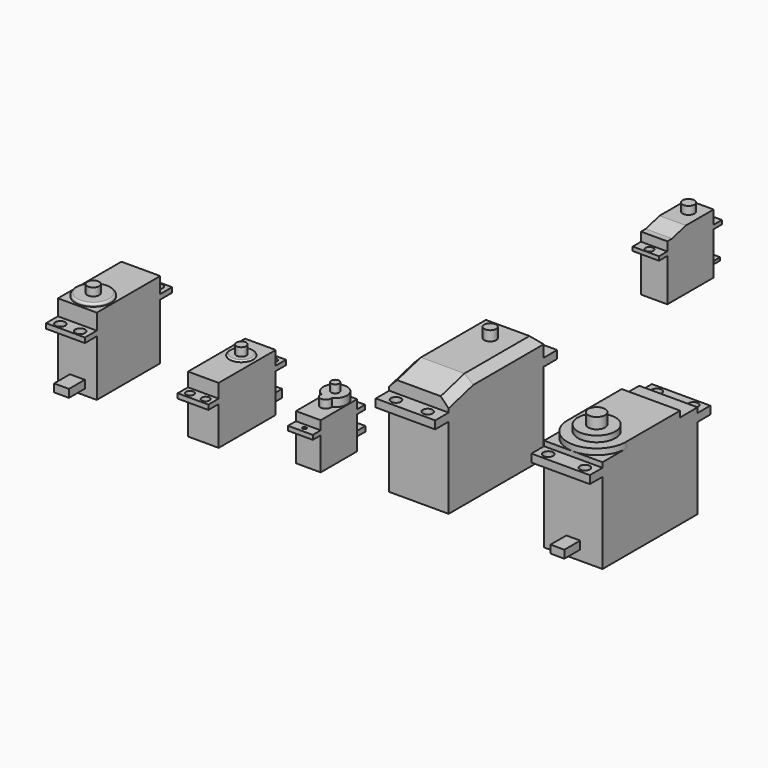
from build123d import *

# Parameters (mm, degrees)
F0_W      = 19.6
F0_H      = 40.05
F1_DEPTH  = 28.3
F2_W      = 19.6
F2_H      = 40.05
F3_DEPTH  = 10.5
F2_H_2    = 7.5
F2_R      = 2.5
F4_DEPTH  = 2.5
F5_R      = 9
F6_DEPTH  = 1.5
F7_R      = 1
F8_R      = 3
F9_DEPTH  = 4
F10_W     = 7.5
F10_H     = 4
F11_DEPTH = 10
F12_W     = 15.5
F12_H     = 36
F13_DEPTH = 19.5
F14_W     = 15.5
F14_H     = 36
F14_H_2   = 6.5
F14_R     = 2
F15_DEPTH = 2.4
F16_W     = 15.5
F16_H     = 36
F17_DEPTH = 7
F18_R     = 6
F19_DEPTH = 0.65
F21_R     = 2.5
F22_DEPTH = 4.2
F23_W     = 6
F23_H     = 4
F24_DEPTH = 10
F25_W     = 12.5
F25_H     = 23
F26_DEPTH = 16.5
F27_W     = 12.5
F27_H     = 5
F27_R     = 1
F27_H_2   = 23
F28_DEPTH = 2.2
F29_W     = 12.5
F29_H     = 23
F30_DEPTH = 4.5
F32_DEPTH = 4
F33_R     = 2
F34_DEPTH = 4
F35_W     = 5
F35_H     = 2.5
F36_DEPTH = 10
F38_DEPTH = 13.3
F39_R     = 3
F40_DEPTH = 4
F41_R     = 2
F42_DEPTH = 34.3511621783
F43_W     = 4
F43_H     = 1.5
F44_DEPTH = 10
F45_W     = 30
F45_H     = 60
F46_DEPTH = 41
F47_W     = 30
F47_H     = 60
F48_DEPTH = 14
F47_H_2   = 8.5
F47_R     = 2.5
F49_DEPTH = 4
F50_R     = 3
F51_DEPTH = 5
F52_SIZE2 = 4
F52_SIZE  = 15
F53_SIZE  = 4
F54_W     = 8
F54_H     = 5
F55_DEPTH = 10
F56_W     = 29.5
F56_H     = 60
F57_DEPTH = 41
F58_W     = 29.5
F58_H     = 60
F59_DEPTH = 6.5
F58_H_2   = 8
F58_R     = 2.5
F60_DEPTH = 4
F62_DEPTH = 3
F63_R     = 9.5
F64_DEPTH = 3
F65_R     = 4.25
F66_DEPTH = 5.5
F67_W     = 7
F67_H     = 4
F68_DEPTH = 10


# Not quite as in the source:
# - a fillet or chamfer that OpenCascade refuses, or shapes differently, is made with other operations: its cross-section is extruded or revolved along the edge and cut away or added


with BuildPart() as f1:
    # F0 (on Top) → F1 (new body)
    with BuildSketch(Plane.XY):
        with Locations((-134.1864168644, -61.3061293165)):
            Rectangle(F0_W, F0_H)
    extrude(amount=F1_DEPTH)

    # F2 (on face) → F3 (join)
    with BuildSketch(Plane.XY.offset(28.3)):
        with Locations((-134.1864168644, -61.3061293165)):
            Rectangle(F2_W, F2_H)
    extrude(amount=F3_DEPTH)

    # F2 (on face) → F4 (join)
    with BuildSketch(Plane.XY.offset(28.3)):
        with Locations((-134.1864168644, -37.5311293165)):
            Rectangle(F2_W, F2_H_2)
        with Locations((-139.1864168644, -36.7811293165)):
            Circle(F2_R, mode=Mode.SUBTRACT)
        with Locations((-129.1864168644, -36.7811293165)):
            Circle(F2_R, mode=Mode.SUBTRACT)
        with Locations((-134.1864168644, -85.0811293165)):
            Rectangle(F2_W, F2_H_2)
        with Locations((-139.1864168644, -85.8311293165)):
            Circle(F2_R, mode=Mode.SUBTRACT)
        with Locations((-129.1864168644, -85.8311293165)):
            Circle(F2_R, mode=Mode.SUBTRACT)
    extrude(amount=F4_DEPTH)

    # F5 (on face) → F6 (join)
    with BuildSketch(Plane.XY.offset(38.8)):
        with Locations((-134.1864168644, -71.3311293165)):
            Circle(F5_R)
    extrude(amount=F6_DEPTH)

    # F7
    f7_edges = [f1.edges().sort_by_distance(p)[0] for p in [
        (-143.186417, -71.331129, 40.3),
    ]]
    fillet(f7_edges, radius=F7_R)

    # F8 (on face) → F9 (join)
    with BuildSketch(Plane.XY.offset(40.3)):
        with Locations((-134.1864168644, -71.3311293165)):
            Circle(F8_R)
    extrude(amount=F9_DEPTH)

    # F10 (on face) → F11 (join)
    with BuildSketch(Plane.XZ.offset(81.3311293165)):
        with Locations((-134.1864168644, 5)):
            Rectangle(F10_W, F10_H)
    extrude(amount=F11_DEPTH)


with BuildPart() as f13:
    # F12 (on Top) → F13 (new body)
    with BuildSketch(Plane.XY):
        with Locations((-69.018992722, -65.2875445485)):
            Rectangle(F12_W, F12_H)
    extrude(amount=F13_DEPTH)

    # F14 (on face) → F15 (join)
    with BuildSketch(Plane.XY.offset(19.5)):
        with Locations((-69.018992722, -65.2875445485)):
            Rectangle(F14_W, F14_H)
        with Locations((-69.018992722, -86.5375445485)):
            Rectangle(F14_W, F14_H_2)
        with Locations((-72.968992722, -86.7875445485)):
            Circle(F14_R, mode=Mode.SUBTRACT)
        with Locations((-65.068992722, -86.7875445485)):
            Circle(F14_R, mode=Mode.SUBTRACT)
        with Locations((-69.018992722, -44.0375445485)):
            Rectangle(F14_W, F14_H_2)
        with Locations((-72.968992722, -44.2875445485)):
            Circle(F14_R, mode=Mode.SUBTRACT)
        with Locations((-65.068992722, -44.2875445485)):
            Circle(F14_R, mode=Mode.SUBTRACT)
    extrude(amount=F15_DEPTH)

    # F16 (on face) → F17 (join)
    with BuildSketch(Plane.XY.offset(21.9)):
        with Locations((-69.018992722, -65.2875445485)):
            Rectangle(F16_W, F16_H)
    extrude(amount=F17_DEPTH)

    # F18 (on face) → F19 (join)
    with BuildSketch(Plane.XY.offset(28.9)):
        with Locations((-69.018992722, -59.2875445485)):
            Circle(F18_R)
    extrude(amount=F19_DEPTH)

    # F20: fillet of radius 1 on 1 edges, made by hand

    # F20_s1 → F20_t2 (revolve, cut)
    with BuildSketch(Plane.XZ.offset(59.2875445485)):
        with BuildLine():
            ThreePointArc((-63.018992722, 28.9), (-63.3856547092, 29.3715838363), (-63.9557424218, 29.55))
            Line((-63.9557424218, 29.55), (-63.018992722, 29.55))
            Line((-63.018992722, 29.55), (-63.018992722, 28.9))
        make_face()
    revolve(axis=Axis((-69.018992722, -59.2875445485, 29.55), (0, 0, 1)), mode=Mode.SUBTRACT)

    # F21 (on face) → F22 (join)
    with BuildSketch(Plane.XY.offset(29.55)):
        with Locations((-69.018992722, -59.2875445485)):
            Circle(F21_R)
    extrude(amount=F22_DEPTH)

    # F23 (on face) → F24 (join)
    with BuildSketch(Plane(origin=(0, -47.2875445485, 0), x_dir=(-1, 0, 0), z_dir=(0, 1, 0))):
        with Locations((69.018992722, 4)):
            Rectangle(F23_W, F23_H)
    extrude(amount=F24_DEPTH)


with BuildPart() as f26:
    # F25 (on Top) → F26 (new body)
    with BuildSketch(Plane.XY):
        with Locations((-23.0503879488, -63.0053216815)):
            Rectangle(F25_W, F25_H)
    extrude(amount=F26_DEPTH)

    # F27 (on face) → F28 (join)
    with BuildSketch(Plane.XY.offset(16.5)):
        with Locations((-23.0503879488, -77.0053216815)):
            Rectangle(F27_W, F27_H)
        with Locations((-23.0503879488, -77.0053216815)):
            Circle(F27_R, mode=Mode.SUBTRACT)
        with Locations((-23.0503879488, -63.0053216815)):
            Rectangle(F27_W, F27_H_2)
        with Locations((-23.0503879488, -49.0053216815)):
            Rectangle(F27_W, F27_H)
        with Locations((-23.0503879488, -49.0053216815)):
            Circle(F27_R, mode=Mode.SUBTRACT)
    extrude(amount=F28_DEPTH)

    # F29 (on face) → F30 (join)
    with BuildSketch(Plane.XY.offset(18.7)):
        with Locations((-23.0503879488, -63.0053216815)):
            Rectangle(F29_W, F29_H)
    extrude(amount=F30_DEPTH)

    # F31 (on face) → F32 (join)
    with BuildSketch(Plane.XY.offset(23.2)):
        with BuildLine():
            ThreePointArc((-25.6349635825, -62.9201133482), (-23.0503879488, -66.1553216815), (-20.465812315, -62.9201133482))
            ThreePointArc((-20.465812315, -62.9201133482), (-17.1985185893, -56.1803216815), (-23.0503879488, -51.5053216815))
            ThreePointArc((-23.0503879488, -51.5053216815), (-28.9022573082, -56.1803216815), (-25.6349635825, -62.9201133482))
        make_face()
    extrude(amount=F32_DEPTH)

    # F33 (on face) → F34 (join)
    with BuildSketch(Plane.XY.offset(27.2)):
        with Locations((-23.0503879488, -57.5053216815)):
            Circle(F33_R)
    extrude(amount=F34_DEPTH)

    # F35 (on face) → F36 (join)
    with BuildSketch(Plane(origin=(0, -51.5053216815, 0), x_dir=(-1, 0, 0), z_dir=(0, 1, 0))):
        with Locations((23.0503879488, 4.75)):
            Rectangle(F35_W, F35_H)
    extrude(amount=F36_DEPTH)


with BuildPart() as f38:
    # F37 (on Right) → F38 (new body)
    with BuildSketch(Plane.YZ):
        Polygon((106.6633449197, 32.3501621783), (106.6633449197, 10.8501621783), (135.8633449197, 10.8501621783), (135.8633449197, 32.3501621783), (141.1133449197, 32.3501621783), (141.1133449197, 34.3501621783), (135.8633449197, 34.3501621783), (135.8633449197, 41.1501621783), (118.3633449197, 41.1501621783), (109.6633449197, 38.8501621783), (106.6633449197, 38.8501621783), (106.6633449197, 34.3501621783), (101.4133449197, 34.3501621783), (101.4133449197, 32.3501621783), align=None)
    extrude(amount=F38_DEPTH)

    # F39 (on face) → F40 (join)
    with BuildSketch(Plane.XY.offset(41.1501621783)):
        with Locations((6.65, 128.3633449197)):
            Circle(F39_R)
    extrude(amount=F40_DEPTH)

    # F41 (on face) → F42 (cut, through all)
    with BuildSketch(Plane.XY.offset(34.3501621783)):
        with Locations((6.65, 103.6633449197)):
            Circle(F41_R)
        with Locations((6.65, 138.8633449197)):
            Circle(F41_R)
    extrude(amount=-F42_DEPTH, mode=Mode.SUBTRACT)

    # F43 (on face) → F44 (join)
    with BuildSketch(Plane(origin=(0, 135.8633449197, 0), x_dir=(-1, 0, 0), z_dir=(0, 1, 0))):
        with Locations((-6.65, 13.6001621783)):
            Rectangle(F43_W, F43_H)
    extrude(amount=F44_DEPTH)


with BuildPart() as f46:
    # F45 (on Top) → F46 (new body)
    with BuildSketch(Plane.XY):
        with Locations((29.7119686007, -40.6373527646)):
            Rectangle(F45_W, F45_H)
    extrude(amount=F46_DEPTH)

    # F47 (on face) → F48 (join)
    with BuildSketch(Plane.XY.offset(41)):
        with Locations((29.7119686007, -40.6373527646)):
            Rectangle(F47_W, F47_H)
    extrude(amount=F48_DEPTH)

    # F47 (on face) → F49 (join)
    with BuildSketch(Plane.XY.offset(41)):
        with Locations((29.7119686007, -74.8873527646)):
            Rectangle(F47_W, F47_H_2)
        with Locations((21.7119686007, -75.1373527646)):
            Circle(F47_R, mode=Mode.SUBTRACT)
        with Locations((37.7119686007, -75.1373527646)):
            Circle(F47_R, mode=Mode.SUBTRACT)
        with Locations((29.7119686007, -6.3873527646)):
            Rectangle(F47_W, F47_H_2)
        with Locations((21.7119686007, -6.1373527646)):
            Circle(F47_R, mode=Mode.SUBTRACT)
        with Locations((37.7119686007, -6.1373527646)):
            Circle(F47_R, mode=Mode.SUBTRACT)
    extrude(amount=F49_DEPTH)

    # F50 (on face) → F51 (join)
    with BuildSketch(Plane.XY.offset(55)):
        with Locations((29.7119686007, -25.6373527646)):
            Circle(F50_R)
    extrude(amount=F51_DEPTH)

    # F52
    f52_edges = [f46.edges().sort_by_distance(p)[0] for p in [
        (29.711969, -70.637353, 55),
    ]]
    f52_side = f46.faces().sort_by_distance((29.711969, -40.876732, 55))[0]
    chamfer(f52_edges, length=F52_SIZE, length2=F52_SIZE2, reference=f52_side)

    # F53
    f53_edges = [f46.edges().sort_by_distance(p)[0] for p in [
        (44.711969, -63.137353, 53),
        (44.711969, -33.137353, 55),
        (29.711969, -10.637353, 55),
        (14.711969, -33.137353, 55),
        (14.711969, -63.137353, 53),
    ]]
    chamfer(f53_edges, length=F53_SIZE)

    # F54 (on face) → F55 (join)
    with BuildSketch(Plane(origin=(0, -10.6373527646, 0), x_dir=(-1, 0, 0), z_dir=(0, 1, 0))):
        with Locations((-29.7119686007, 6.5)):
            Rectangle(F54_W, F54_H)
    extrude(amount=F55_DEPTH)


with BuildPart() as f57:
    # F56 (on Top) → F57 (new body)
    with BuildSketch(Plane.XY):
        with Locations((106.7800781727, -39.5376843214)):
            Rectangle(F56_W, F56_H)
    extrude(amount=F57_DEPTH)

    # F58 (on face) → F59 (join)
    with BuildSketch(Plane.XY.offset(41)):
        with Locations((106.7800781727, -39.5376843214)):
            Rectangle(F58_W, F58_H)
    extrude(amount=F59_DEPTH)

    # F58 (on face) → F60 (join)
    with BuildSketch(Plane.XY.offset(41)):
        with Locations((106.7800781727, -73.5376843214)):
            Rectangle(F58_W, F58_H_2)
        with Locations((97.5300781727, -73.7876843214)):
            Circle(F58_R, mode=Mode.SUBTRACT)
        with Locations((116.0300781727, -73.7876843214)):
            Circle(F58_R, mode=Mode.SUBTRACT)
        with Locations((106.7800781727, -5.5376843214)):
            Rectangle(F58_W, F58_H_2)
        with Locations((97.5300781727, -5.2876843214)):
            Circle(F58_R, mode=Mode.SUBTRACT)
        with Locations((116.0300781727, -5.2876843214)):
            Circle(F58_R, mode=Mode.SUBTRACT)
    extrude(amount=F60_DEPTH)

    # F61 (on face) → F62 (join)
    with BuildSketch(Plane.XY.offset(47.5)):
        with BuildLine():
            Line((92.0300781727, -20.5376843214), (92.0300781727, -54.7876843214))
            ThreePointArc((92.0300781727, -54.7876843214), (96.3502531502, -65.2175093439), (106.7800781727, -69.5376843214))
            ThreePointArc((106.7800781727, -69.5376843214), (117.2099031952, -65.2175093439), (121.5300781727, -54.7876843214))
            Line((121.5300781727, -54.7876843214), (121.5300781727, -20.5376843214))
            Line((121.5300781727, -20.5376843214), (92.0300781727, -20.5376843214))
        make_face()
    extrude(amount=F62_DEPTH)

    # F63 (on face) → F64 (join)
    with BuildSketch(Plane.XY.offset(50.5)):
        with Locations((106.7800781727, -54.7876843214)):
            Circle(F63_R)
    extrude(amount=F64_DEPTH)

    # F65 (on face) → F66 (join)
    with BuildSketch(Plane.XY.offset(53.5)):
        with Locations((106.7800781727, -54.7876843214)):
            Circle(F65_R)
    extrude(amount=F66_DEPTH)

    # F67 (on face) → F68 (join)
    with BuildSketch(Plane.XZ.offset(69.5376843214)):
        with Locations((106.7800781727, 7)):
            Rectangle(F67_W, F67_H)
    extrude(amount=F68_DEPTH)


solid = Compound([f1.part, f13.part, f26.part, f38.part, f46.part, f57.part])
